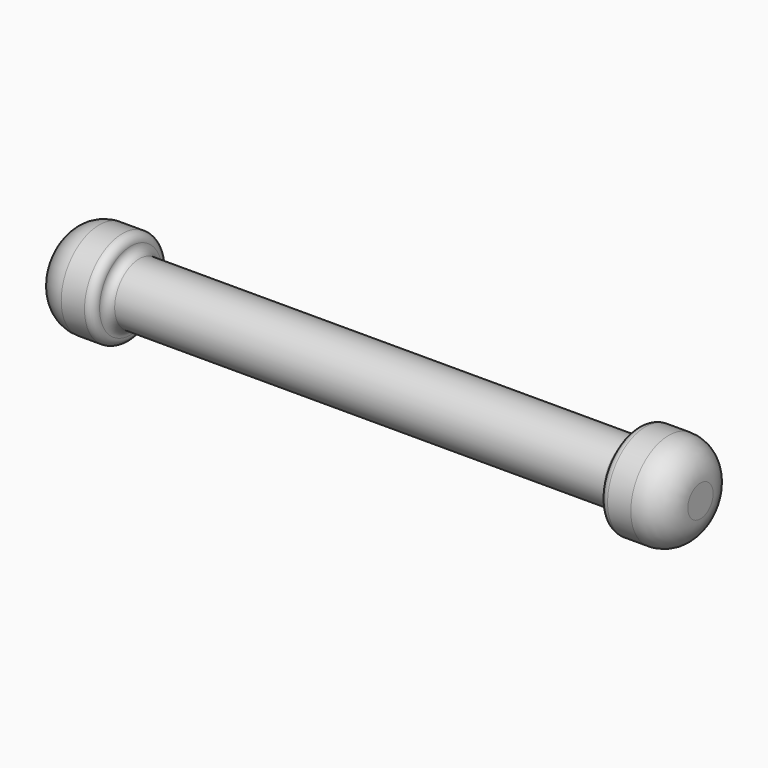
from build123d import *

# Parameters (mm, degrees)
F0_R     = 4.85
F1_DEPTH = 80
F2_R     = 7.5
F3_DEPTH = 10
F4_R     = 7.5
F5_DEPTH = 10
F6_R     = 1.32499
F7_R     = 1.32499
F8_R     = 5


# Not quite as in the source:
# - a fillet or chamfer is up to 0.001 mm smaller than in the source, because OpenCascade refuses the exact size


with BuildPart() as f1:
    # F0 (on Right) → F1 (new body)
    with BuildSketch(Plane.YZ):
        Circle(F0_R)
    extrude(amount=F1_DEPTH)

    # F2 (on face) → F3 (join)
    with BuildSketch(Plane.YZ.offset(80)):
        Circle(F2_R)
    extrude(amount=F3_DEPTH)

    # F4 (on face) → F5 (join)
    with BuildSketch(Plane(origin=(0, 0, 0), x_dir=(0, -1, 0), z_dir=(-1, 0, 0))):
        Circle(F4_R)
    extrude(amount=F5_DEPTH)

    # F6 (radius 1.325 in the source; OpenCascade refuses exactly that, so slightly less here)
    f6_edges = [f1.edges().sort_by_distance(p)[0] for p in [
        (0, -4.85, 0),
        (0, 7.5, 0),
    ]]
    fillet(f6_edges, radius=F6_R)

    # F7 (radius 1.325 in the source; OpenCascade refuses exactly that, so slightly less here)
    f7_edges = [f1.edges().sort_by_distance(p)[0] for p in [
        (80, -4.85, 0),
        (80, -7.5, 0),
    ]]
    fillet(f7_edges, radius=F7_R)

    # F8
    f8_edges = [f1.edges().sort_by_distance(p)[0] for p in [
        (-10, 7.5, 0),
        (90, -7.5, 0),
    ]]
    fillet(f8_edges, radius=F8_R)


solid = f1.part
